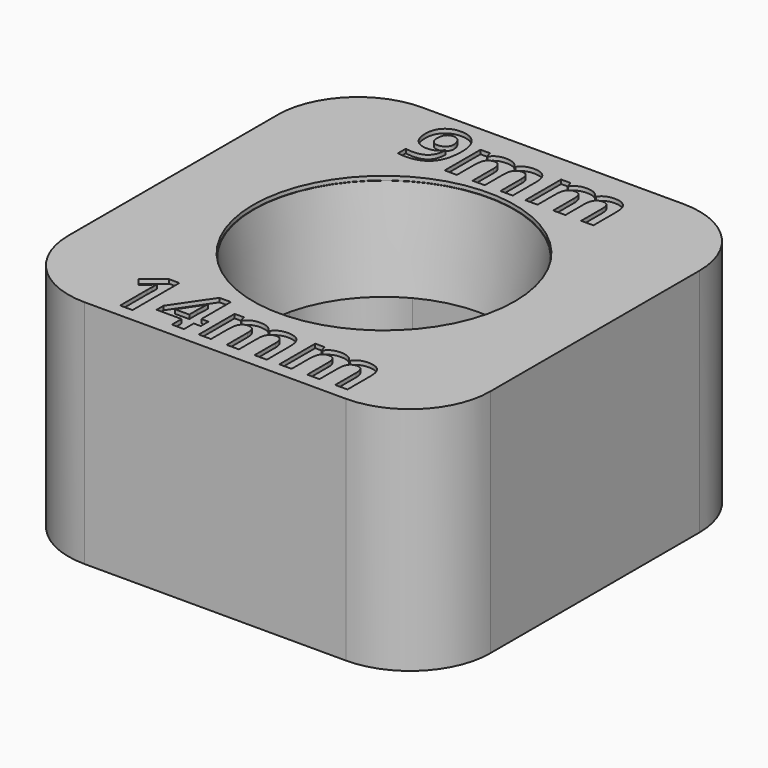
from build123d import *

# Parameters (mm, degrees)
F0_W           = 42.1
F0_H           = 42.1
F0_R           = 13.05
F1_DEPTH       = 23
F2_R           = 10.25
F5_R           = 8
F6_T           = -1.2
F7_R           = 13.05
F7_TEXT_SIZE   = 8.1944444444
F7_TEXT_SIZE_2 = 8.1972222222
F8_DEPTH       = 0.4
F9_W           = 28.1658135355
F9_H           = 29.1879680008
F10_DEPTH      = 13


# Not quite as in the source:
# - Text() gives the source's letters only with a copy of the font that has no kerning and outlines rounded to 1/6400 em; it was checked with that copy


with BuildPart() as f1:
    # F0 (on Top) → F1 (new body)
    with BuildSketch(Plane.XY):
        Rectangle(F0_W, F0_H)
        Circle(F0_R, mode=Mode.SUBTRACT)
        Circle(F0_R)
    extrude(amount=-F1_DEPTH)


with BuildPart() as f3:
    # F0 (on Top) → F3 section 0
    with BuildSketch(Plane.XY):
        Circle(F0_R)
    # F2 (on face) → F3 section 1
    with BuildSketch(Plane(origin=(0, 0, -23), x_dir=(1, 0, 0), z_dir=(0, 0, -1))):
        Circle(F2_R)
    loft()


with BuildPart() as f1_1:
    add(f1.part)

    # F4: cut F3
    add(f3.part, mode=Mode.SUBTRACT)

    # F5
    f5_edges = [f1_1.edges().sort_by_distance(p)[0] for p in [
        (-21.05, -21.05, -11.5),
        (-21.05, 21.05, -11.5),
        (21.05, 21.05, -11.5),
        (21.05, -21.05, -11.5),
    ]]
    fillet(f5_edges, radius=F5_R)

    # F6
    f6_openings = [f1_1.faces().sort_by_distance(p)[0] for p in [
        (0, -20.454616, -23),
    ]]
    offset(amount=F6_T, openings=f6_openings, kind=Kind.INTERSECTION)

    # F7 (on face) → F8 (cut)
    with BuildSketch(Plane.XY):
        Circle(F7_R)
        with Locations((-12.6828233507, -19.75)):
            Text('14mm', F7_TEXT_SIZE, font='Open Sans', font_style=FontStyle.BOLD, text_align=(TextAlign.LEFT, TextAlign.BOTTOM))
        with Locations((-10.3477122396, 13.85)):
            Text('9mm', F7_TEXT_SIZE_2, font='Open Sans', font_style=FontStyle.BOLD, text_align=(TextAlign.LEFT, TextAlign.BOTTOM))
    extrude(amount=-F8_DEPTH, mode=Mode.SUBTRACT)

    # F9 (on face) → F10 (cut)
    with BuildSketch(Plane(origin=(0, 0, -23), x_dir=(1, 0, 0), z_dir=(0, 0, -1))):
        Rectangle(F9_W, F9_H)
    extrude(amount=-F10_DEPTH, mode=Mode.SUBTRACT)


solid = f1_1.part
